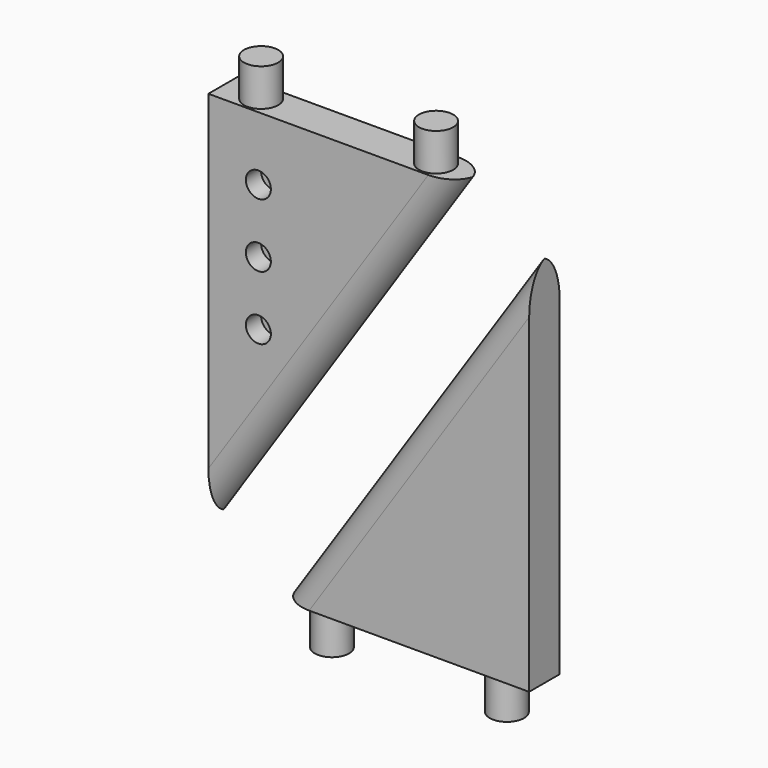
from build123d import *

# Parameters (mm, degrees)
F1_DEPTH      = 7.62
F2_R          = 3.429
F4_DEPTH      = 7.5
F3_R          = 3.429
F5_DEPTH      = 7.5
F6_T1_DEPTH   = 115.1387818866
F6_2_T1_DEPTH = 115.1387818866
F7_R          = 2.5
F9_DEPTH      = 3.81
F8_R          = 2.5
F10_DEPTH     = 3.81


# Not quite as in the source:
# - a fillet or chamfer that OpenCascade refuses, or shapes differently, is made with other operations: its cross-section is extruded or revolved along the edge and cut away or added


with BuildPart() as f1:
    # F0 (on Front) → F1 (new body)
    with BuildSketch(Plane.XZ):
        Polygon((25, 37.5), (-25, -37.5), (25, -37.5), align=None)
    extrude(amount=F1_DEPTH)

    # F3 (on face) → F5 (join)
    with BuildSketch(Plane(origin=(0, 0, -37.5), x_dir=(1, 0, 0), z_dir=(0, 0, -1))):
        with Locations((-17.5, 3.81)):
            Circle(F3_R)
        with Locations((17.5, 3.81)):
            Circle(F3_R)
    extrude(amount=F5_DEPTH)

    # F6: fillet of radius 5 on 2 edges, made by hand

    # F6_s2 → F6_t1 (cut)
    with BuildSketch(Plane(origin=(31.9337524528, 0, 47.9006286792), x_dir=(0, 1, 0), z_dir=(-0.5547001962, 0, -0.8320502943))):
        with BuildLine():
            ThreePointArc((-2.62, 0), (-6.1555339059, 1.4644660941), (-7.62, 5))
            Line((-7.62, 5), (-7.62, 0))
            Line((-7.62, 0), (-2.62, 0))
        make_face()
        with BuildLine():
            ThreePointArc((-5, 0), (-1.4644660941, 1.4644660941), (0, 5))
            Line((0, 5), (0, 0))
            Line((0, 0), (-5, 0))
        make_face()
    extrude(amount=F6_T1_DEPTH, mode=Mode.SUBTRACT)

    # F7 (on face) → F9 (cut)
    with BuildSketch(Plane(origin=(0, 0, 0), x_dir=(-1, 0, 0), z_dir=(0, 1, 0))):
        with Locations((-15, -24.7534695472)):
            Circle(F7_R)
        with Locations((-15, -12.0069390943)):
            Circle(F7_R)
        with Locations((-15, 0.7395913585)):
            Circle(F7_R)
    extrude(amount=-F9_DEPTH, mode=Mode.SUBTRACT)


with BuildPart() as f1b:
    # F0 (on Front) → F1, piece 2 (new body)
    with BuildSketch(Plane.XZ):
        Polygon((-39.1634743611, -28.0576837592), (10.8365256389, 46.9423162408), (-39.1634743611, 46.9423162408), align=None)
    extrude(amount=F1_DEPTH)

    # F2 (on face) → F4 (join)
    with BuildSketch(Plane.XY.offset(46.9423162408)):
        with Locations((-31.6634743611, -3.81)):
            Circle(F2_R)
        with Locations((3.3365256389, -3.81)):
            Circle(F2_R)
    extrude(amount=F4_DEPTH)

    # F6#2: fillet of radius 5 on 2 edges, made by hand

    # F6_2_s2 → F6_2_t1 (cut)
    with BuildSketch(Plane(origin=(-31.9337524528, 0, -47.9006286792), x_dir=(0, 1, 0), z_dir=(0.5547001962, 0, 0.8320502943))):
        with BuildLine():
            ThreePointArc((-5, 17.0223776826), (-1.4644660941, 18.4868437767), (0, 22.0223776826))
            Line((0, 22.0223776826), (0, 17.0223776826))
            Line((0, 17.0223776826), (-5, 17.0223776826))
        make_face()
        with BuildLine():
            ThreePointArc((-2.62, 17.0223776826), (-6.1555339059, 18.4868437767), (-7.62, 22.0223776826))
            Line((-7.62, 22.0223776826), (-7.62, 17.0223776826))
            Line((-7.62, 17.0223776826), (-2.62, 17.0223776826))
        make_face()
    extrude(amount=F6_2_T1_DEPTH, mode=Mode.SUBTRACT)

    # F8 (on face) → F10 (cut)
    with BuildSketch(Plane.XZ.offset(7.62)):
        with Locations((-29.1634743611, 8.7027248823)):
            Circle(F8_R)
        with Locations((-29.1634743611, 21.4492553351)):
            Circle(F8_R)
        with Locations((-29.1634743611, 34.1957857879)):
            Circle(F8_R)
    extrude(amount=-F10_DEPTH, mode=Mode.SUBTRACT)


solid = Compound([f1.part, f1b.part])
